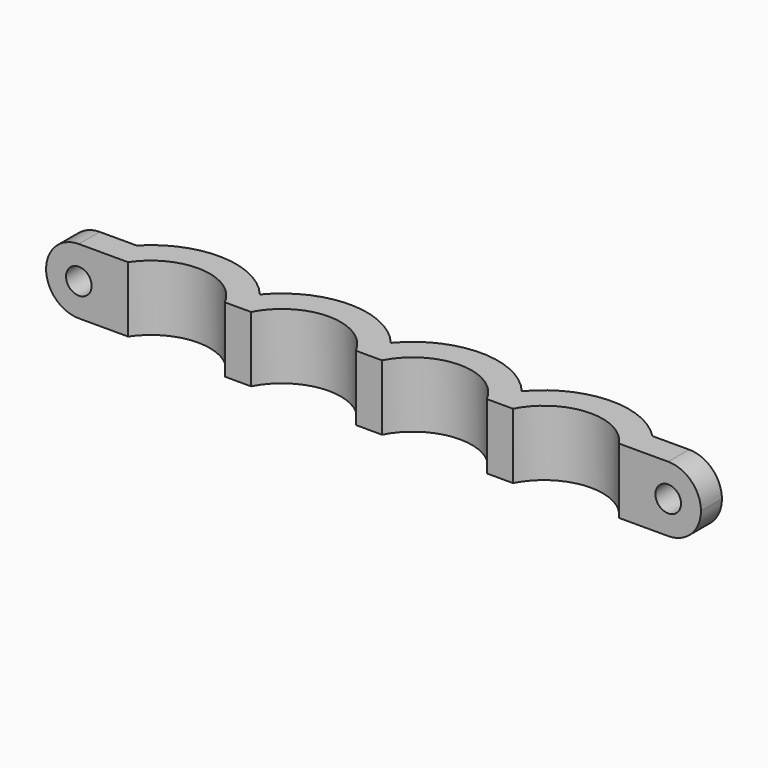
from build123d import *

# Parameters (mm, degrees)
F1_DEPTH = 7.9375
F2_R     = 1.5512489022
F3_DEPTH = 3.175
F4_R     = 3.175
F5_DEPTH = 25.4
F6_R     = 3.96874


# Not quite as in the source:
# - a fillet or chamfer is up to 0.001 mm smaller than in the source, because OpenCascade refuses the exact size


with BuildPart() as f1:
    # F0 (on Top) → F1 (new body)
    with BuildSketch(Plane.XY):
        with BuildLine():
            Line((-9.9351188985, 0), (0, 0))
            ThreePointArc((0, 0), (6.3438186296, 3.1635706978), (12.2898811015, -0.6960349097))
            Line((12.2898811015, -0.6960349097), (15.4648811015, -0.6960349097))
            ThreePointArc((15.4648811015, -0.6960349097), (21.8148811015, 3.175), (28.1648811015, -0.6960349097))
            Line((28.1648811015, -0.6960349097), (31.3398811015, -0.6960349097))
            ThreePointArc((31.3398811015, -0.6960349097), (37.6898811015, 3.175), (44.0398811015, -0.6960349097))
            Line((44.0398811015, -0.6960349097), (47.2148811015, -0.6960349097))
            ThreePointArc((47.2148811015, -0.6960349097), (53.1609435734, 3.1635706978), (59.504762203, 0))
            Line((59.504762203, 0), (69.4398811015, 0))
            Line((69.4398811015, 0), (69.4398811015, 3.175))
            Line((69.4398811015, 3.175), (61.0109161202, 3.175))
            ThreePointArc((61.0109161202, 3.175), (53.1959495352, 6.3434025911), (45.6273811015, 2.6246326912))
            ThreePointArc((45.6273811015, 2.6246326912), (37.6898811015, 6.35), (29.7523811015, 2.6246326912))
            ThreePointArc((29.7523811015, 2.6246326912), (21.8148811015, 6.35), (13.8773811015, 2.6246326912))
            ThreePointArc((13.8773811015, 2.6246326912), (6.3088126678, 6.3434025911), (-1.5061539172, 3.175))
            Line((-1.5061539172, 3.175), (-9.9351188985, 3.175))
            Line((-9.9351188985, 3.175), (-9.9351188985, 0))
        make_face()
    extrude(amount=F1_DEPTH)

    # F2 (on face) → F3 (cut, through all)
    with BuildSketch(Plane(origin=(0, 3.175, 0), x_dir=(-1, 0, 0), z_dir=(0, 1, 0))):
        with Locations((5.9663688985, 3.96875)):
            Circle(F2_R)
        with Locations((-65.4711311015, 3.96875)):
            Circle(F2_R)
    extrude(amount=-F3_DEPTH, mode=Mode.SUBTRACT)

    # F4 (on face) → F5 (cut)
    with BuildSketch(Plane(origin=(0, 3.175, 0), x_dir=(-1, 0, 0), z_dir=(0, 1, 0))):
        with Locations((5.9663688985, 3.96875)):
            Circle(F4_R)
        with Locations((-65.4711311015, 3.96875)):
            Circle(F4_R)
    extrude(amount=F5_DEPTH, mode=Mode.SUBTRACT)

    # F6 (radius 3.96875 in the source; OpenCascade refuses exactly that, so slightly less here)
    f6_edges = [f1.edges().sort_by_distance(p)[0] for p in [
        (69.439881, 1.5875, 7.9375),
        (69.439881, 1.5875, 0),
        (-9.935119, 1.5875, 7.9375),
        (-9.935119, 1.5875, 0),
    ]]
    fillet(f6_edges, radius=F6_R)


solid = f1.part
